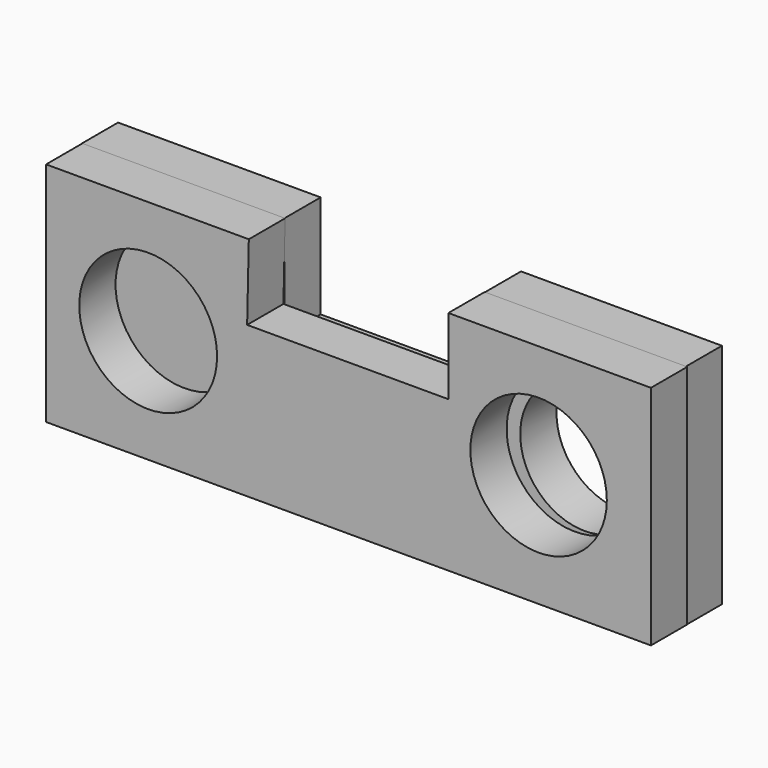
from build123d import *

# Parameters (mm, degrees)
F2_DEPTH  = 18
F0_W      = 80
F0_H      = 47.1640562918
F0_H_2    = 42.8359437082
F0_H_3    = 45
F4_DEPTH  = 25
F5_R      = 27.3467975621
F5_R_2    = 27.0757536819
F6_DEPTH  = 58.2
F8_DEPTH  = 18
F9_R      = 25.5810591855
F10_DEPTH = 63.8


# Not quite as in the source:
# - a feature names something its author has since deleted; it is built from what else it names


with BuildPart() as f2:
    # F1 (on face) → F2 (new body)
    with BuildSketch(Plane.XZ):
        Polygon((39.6220497787, 45.2090576291), (-39.5539887249, 45.2090576291), (-40.2230843902, 14.8768285289), (39.6220497787, 14.8768285289), align=None)
    extrude(amount=F2_DEPTH)


with BuildPart() as f2b:
    # F0 (on Front) → F2, piece 2 (new body)
    with BuildSketch(Plane.XZ):
        with Locations((-80, -21.4179718541)):
            Rectangle(F0_W, F0_H)
        Polygon((-40, 2.1640562918), (-40, -45), (40, -45), (40, 0), (40, 45), (-40, 45), align=None)
        with Locations((-80, 23.5820281459)):
            Rectangle(F0_W, F0_H_2)
        with Locations((80, -22.5)):
            Rectangle(F0_W, F0_H_3)
        with Locations((80, 22.5)):
            Rectangle(F0_W, F0_H_3)
    extrude(amount=F2_DEPTH)


with BuildPart() as f4_tool:
    # F3 (on face) → F4 (new body)
    with BuildSketch(Plane.XZ.offset(18)):
        Polygon((39.6220497787, 14.8768285289), (39.6220497787, 45.2090576291), (-39.5539887249, 45.2090576291), (-40.2230843902, 14.8768285289), align=None)
    extrude(amount=-F4_DEPTH)


with BuildPart() as f2_1:
    add(f2.part)

    # F4: cut by f4_tool
    add(f4_tool.part, mode=Mode.SUBTRACT)


with BuildPart() as f2b_1:
    add(f2b.part)

    # F4: cut by f4_tool
    add(f4_tool.part, mode=Mode.SUBTRACT)

    # F5 (on Front) → F6 (cut)
    with BuildSketch(Plane.XZ):
        with Locations((-79.4878825545, 0)):
            Circle(F5_R)
        with Locations((75.41680336, 0)):
            Circle(F5_R_2)
    extrude(amount=F6_DEPTH, mode=Mode.SUBTRACT)

    # F7 (on Front) → F8 (join)
    with BuildSketch(Plane.XZ):
        Polygon((119.3632781506, -45.4373732209), (119.3632781506, 44.861137867), (39.6516397595, 44.9020341039), (39.6516397595, 4.0344810113), (-39.8564524949, 4.0344810113), (-39.8564524949, 44.9020341039), (-120.2343702316, 44.9020341039), (-120.2343702316, -45.4373732209), align=None)
    extrude(amount=-F8_DEPTH)

    # F9 (on Front) → F10 (cut)
    with BuildSketch(Plane.XZ):
        with Locations((79.3142113835, 0)):
            Circle(F9_R)
    extrude(amount=-F10_DEPTH, mode=Mode.SUBTRACT)


solid = f2b_1.part
